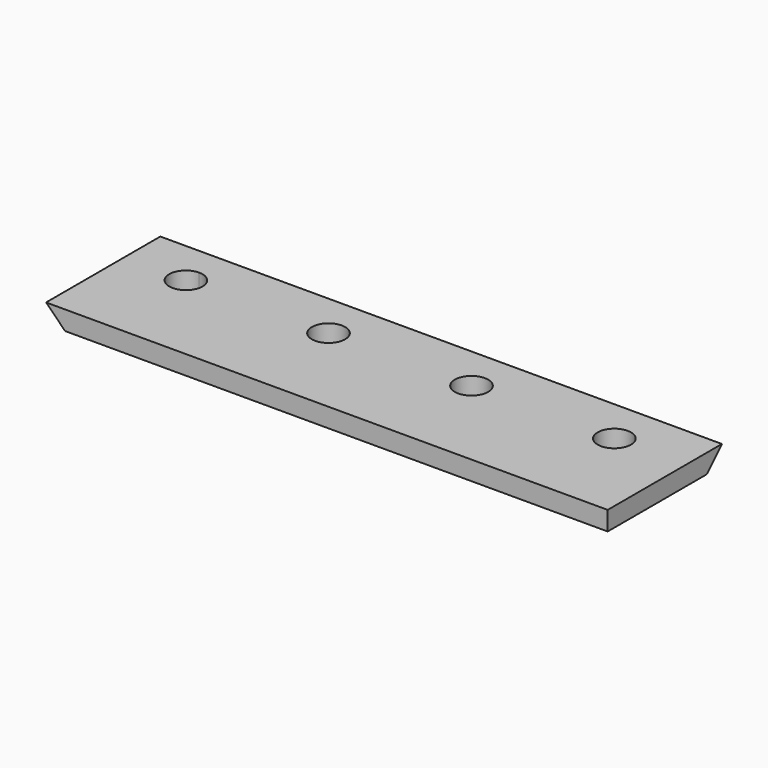
from build123d import *

# Parameters (mm, degrees)
F0_R     = 3.5
F1_DEPTH = 4
F2_SIZE  = 3.99999


# Not quite as in the source:
# - a fillet or chamfer is up to 0.001 mm smaller than in the source, because OpenCascade refuses the exact size


with BuildPart() as f1:
    # F0 (on Top) → F1 (new body)
    with BuildSketch(Plane.XY):
        with BuildLine():
            Line((-58.7463706657, 0.847793646), (-71.7463706657, 0.847793646))
            Line((-71.7463706657, 0.847793646), (-71.7463706657, -3.152206354))
            Line((-71.7463706657, -3.152206354), (-71.7463706657, -5.152206354))
            Line((-71.7463706657, -5.152206354), (-71.7463706657, -29.152206354))
            Line((-71.7463706657, -29.152206354), (-58.7463706657, -29.152206354))
            Line((-58.7463706657, -29.152206354), (-58.7463706657, -12.1857047902))
            ThreePointArc((-58.7463706657, -12.1857047902), (-62.2463706657, -8.6857047902), (-58.7463706657, -5.1857047902))
            Line((-58.7463706657, -5.1857047902), (-58.7463706657, 0.847793646))
        make_face()
        with BuildLine():
            Line((46.2536293343, 0.847793646), (-58.7463706657, 0.847793646))
            Line((-58.7463706657, 0.847793646), (-58.7463706657, -5.1857047902))
            ThreePointArc((-58.7463706657, -5.1857047902), (-56.2714969316, -6.2108310561), (-55.2463706657, -8.6857047902))
            ThreePointArc((-55.2463706657, -8.6857047902), (-56.2714969316, -11.1605785244), (-58.7463706657, -12.1857047902))
            Line((-58.7463706657, -12.1857047902), (-58.7463706657, -29.152206354))
            Line((-58.7463706657, -29.152206354), (46.2536293343, -29.152206354))
            Line((46.2536293343, -29.152206354), (46.2536293343, 0.847793646))
        make_face()
        with Locations((-28.7463706657, -8.7296278255)):
            Circle(F0_R, mode=Mode.SUBTRACT)
        with Locations((1.2536293343, -8.6778136941)):
            Circle(F0_R, mode=Mode.SUBTRACT)
        with Locations((31.2536293343, -8.6667486506)):
            Circle(F0_R, mode=Mode.SUBTRACT)
    extrude(amount=F1_DEPTH)

    # F2 (size 4 in the source; OpenCascade refuses exactly that, so slightly less here)
    f2_edges = [f1.edges().sort_by_distance(p)[0] for p in [
        (-71.746371, -14.152206, 0),
        (-12.746371, 0.847794, 0),
    ]]
    chamfer(f2_edges, length=F2_SIZE)


solid = f1.part
